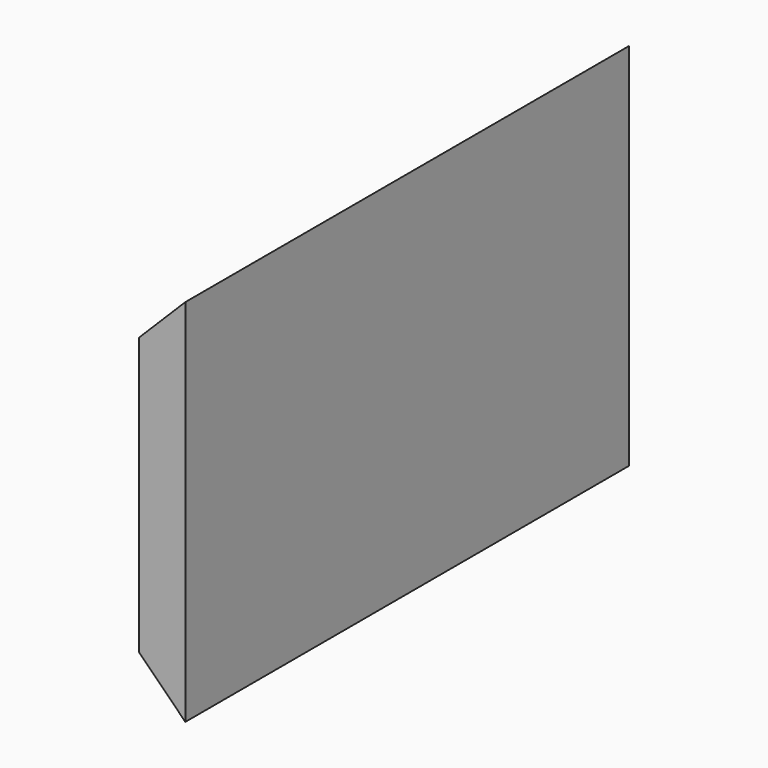
from build123d import *

# Parameters (mm, degrees)
F0_W     = 25
F0_H     = 200
F1_DEPTH = 300
F2_SIZE  = 24.99999
F3_SIZE  = 24.99999


# Not quite as in the source:
# - a fillet or chamfer is up to 0.001 mm smaller than in the source, because OpenCascade refuses the exact size


with BuildPart() as f1:
    # F0 (on Front) → F1 (new body)
    with BuildSketch(Plane.XZ):
        with Locations((12.5, 100)):
            Rectangle(F0_W, F0_H)
    extrude(amount=F1_DEPTH)

    # F2 (size 25 in the source; OpenCascade refuses exactly that, so slightly less here)
    f2_edges = [f1.edges().sort_by_distance(p)[0] for p in [
        (0, -150, 200),
    ]]
    chamfer(f2_edges, length=F2_SIZE)

    # F3 (size 25 in the source; OpenCascade refuses exactly that, so slightly less here)
    f3_edges = [f1.edges().sort_by_distance(p)[0] for p in [
        (0, -150, 0),
    ]]
    chamfer(f3_edges, length=F3_SIZE)


solid = f1.part
